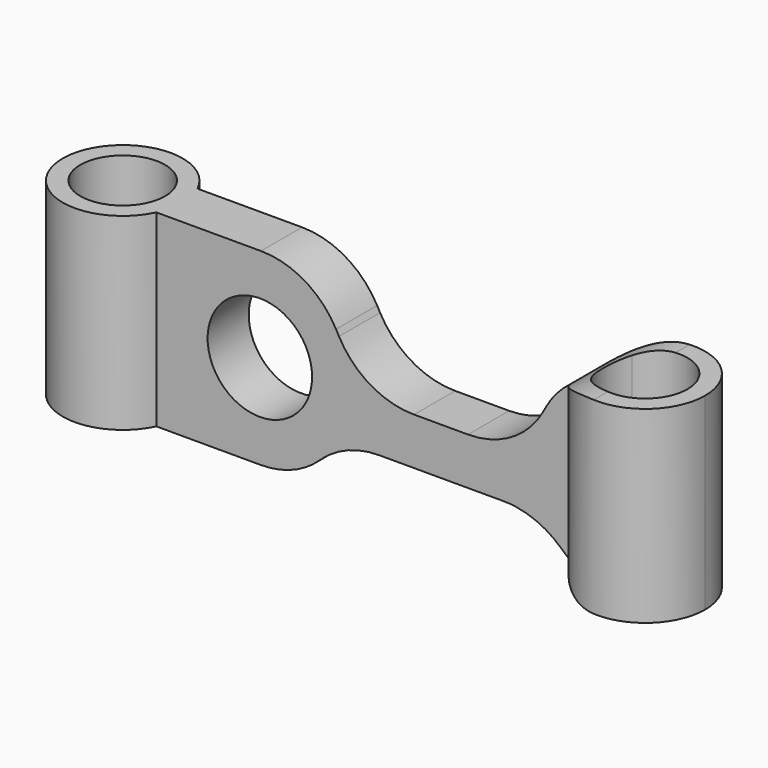
from build123d import *

# Parameters (mm, degrees)
F1_DEPTH    = 11
F2_R        = 3.05
F3_DEPTH    = 3
F4_T1_DEPTH = 3
F4_T3_DEPTH = 17.7890113567
F5_R        = 5


# Not quite as in the source:
# - a fillet or chamfer that OpenCascade refuses, or shapes differently, is made with other operations: its cross-section is extruded or revolved along the edge and cut away or added


with BuildPart() as f1:
    # F0 (on Top) → F1 (new body)
    with BuildSketch(Plane.XY):
        with BuildLine():
            ThreePointArc((13.2813392877, 14.1006531194), (16.0415774558, 14.9456542135), (17.725, 12.6006531194))
            ThreePointArc((17.725, 12.6006531194), (16.0415774558, 10.2556520253), (13.2813392877, 11.1006531194))
            Line((13.2813392877, 11.1006531194), (12.0877223398, 11.1006531194))
            ThreePointArc((12.0877223398, 11.1006531194), (16.0187744108, 9.1861273975), (18.75, 12.6006531194))
            ThreePointArc((18.75, 12.6006531194), (16.0187744108, 16.0151788413), (12.0877223398, 14.1006531194))
            Line((12.0877223398, 14.1006531194), (13.2813392877, 14.1006531194))
        make_face()
        with BuildLine():
            ThreePointArc((13.2813392877, 11.1006531194), (12.775, 12.6006531194), (13.2813392877, 14.1006531194))
            Line((13.2813392877, 14.1006531194), (12.0877223398, 14.1006531194))
            ThreePointArc((12.0877223398, 14.1006531194), (11.75, 12.6006531194), (12.0877223398, 11.1006531194))
            Line((12.0877223398, 11.1006531194), (13.2813392877, 11.1006531194))
        make_face()
        with BuildLine():
            ThreePointArc((12.0877223398, 11.1006531194), (11.75, 12.6006531194), (12.0877223398, 14.1006531194))
            Line((12.0877223398, 14.1006531194), (-12.0877223398, 14.1006531194))
            ThreePointArc((-12.0877223398, 14.1006531194), (-11.8354742781, 13.3694275302), (-11.75, 12.6006531194))
            ThreePointArc((-11.75, 12.6006531194), (-11.8354742781, 11.8318787086), (-12.0877223398, 11.1006531194))
            Line((-12.0877223398, 11.1006531194), (12.0877223398, 11.1006531194))
        make_face()
        with BuildLine():
            ThreePointArc((-11.75, 12.6006531194), (-11.8354742781, 13.3694275302), (-12.0877223398, 14.1006531194))
            Line((-12.0877223398, 14.1006531194), (-13.2813392877, 14.1006531194))
            ThreePointArc((-13.2813392877, 14.1006531194), (-12.9049989059, 13.3922305752), (-12.775, 12.6006531194))
            ThreePointArc((-12.775, 12.6006531194), (-12.9049989059, 11.8090756636), (-13.2813392877, 11.1006531194))
            Line((-13.2813392877, 11.1006531194), (-12.0877223398, 11.1006531194))
            ThreePointArc((-12.0877223398, 11.1006531194), (-11.8354742781, 11.8318787086), (-11.75, 12.6006531194))
        make_face()
        with BuildLine():
            Line((-13.2813392877, 14.1006531194), (-12.0877223398, 14.1006531194))
            ThreePointArc((-12.0877223398, 14.1006531194), (-18.75, 12.6006531194), (-12.0877223398, 11.1006531194))
            Line((-12.0877223398, 11.1006531194), (-13.2813392877, 11.1006531194))
            ThreePointArc((-13.2813392877, 11.1006531194), (-17.725, 12.6006531194), (-13.2813392877, 14.1006531194))
        make_face()
    extrude(amount=F1_DEPTH)

    # F2 (on face) → F3 (cut, through all)
    with BuildSketch(Plane.XZ.offset(-11.1006531194)):
        with Locations((-6.0438611699, 5.5)):
            Circle(F2_R)
        Polygon((12.0877223398, 11), (-3.021930585, 11), (0, 5.5), (9.0657917549, 5.5), align=None)
        Polygon((10.5767570474, 2.75), (-1.5109652925, 2.75), (-3.021930585, 0), (12.0877223398, 0), align=None)
    extrude(amount=-F3_DEPTH, mode=Mode.SUBTRACT)

    # F4: fillet of radius 5 on 6 edges, made by hand

    # F4_s2 → F4_t1 (join)
    with BuildSketch(Plane.XZ.offset(-14.1006531194)):
        with BuildLine():
            ThreePointArc((2.9578022713, 5.5), (0.4120783796, 6.1965955492), (-1.4243095392, 8.0922840533))
            Line((-1.4243095392, 8.0922840533), (0, 5.5))
            Line((0, 5.5), (2.9578022713, 5.5))
        make_face()
        with BuildLine():
            ThreePointArc((10.4901012941, 8.0922840533), (8.6537133753, 6.1965955492), (6.1079894835, 5.5))
            Line((6.1079894835, 5.5), (9.0657917549, 5.5))
            Line((9.0657917549, 5.5), (10.4901012941, 8.0922840533))
        make_face()
    extrude(amount=F4_T1_DEPTH)

    # F4_s4 → F4_t3 (cut)
    with BuildSketch(Plane.XZ.offset(-21.4951587977)):
        with BuildLine():
            ThreePointArc((-1.5976210458, 8.4077159467), (-3.4340089645, 10.3034044508), (-5.9797328563, 11))
            Line((-5.9797328563, 11), (-3.021930585, 11))
            Line((-3.021930585, 11), (-1.5976210458, 8.4077159467))
        make_face()
        with BuildLine():
            ThreePointArc((-5.9797328563, 0), (-3.4340089645, 0.6965955492), (-1.5976210458, 2.5922840533))
            Line((-1.5976210458, 2.5922840533), (-3.021930585, 0))
            Line((-3.021930585, 0), (-5.9797328563, 0))
        make_face()
        with BuildLine():
            ThreePointArc((15.0455246112, 0), (12.4998007194, 0.6965955492), (10.6634128006, 2.5922840533))
            Line((10.6634128006, 2.5922840533), (12.0877223398, 0))
            Line((12.0877223398, 0), (15.0455246112, 0))
        make_face()
        with BuildLine():
            ThreePointArc((15.0455246112, 11), (12.4998007194, 10.3034044508), (10.6634128006, 8.4077159467))
            Line((10.6634128006, 8.4077159467), (12.0877223398, 11))
            Line((12.0877223398, 11), (15.0455246112, 11))
        make_face()
    extrude(amount=F4_T3_DEPTH, mode=Mode.SUBTRACT)

    # F5
    f5_edges = [f1.edges().sort_by_distance(p)[0] for p in [
        (10.576757, 12.600653, 2.75),
        (-1.510965, 12.600653, 2.75),
    ]]
    fillet(f5_edges, radius=F5_R)


solid = f1.part
